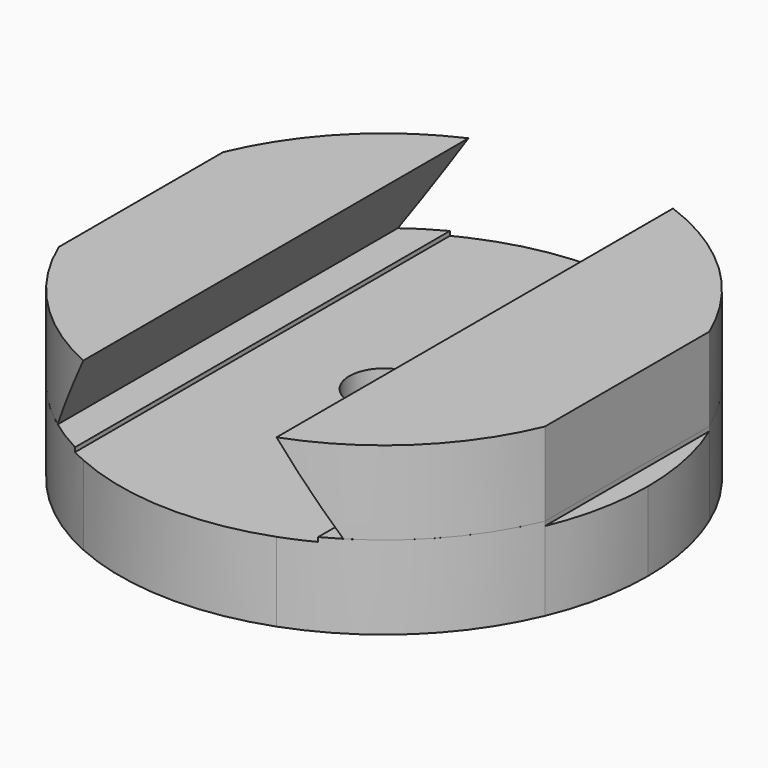
from build123d import *

# Parameters (mm, degrees)
F0_W          = 98.044
F0_H          = 98.044
F1_DEPTH      = 15.24
F3_D          = 12.7
F2_W          = 4.572
F2_H          = 98.044
F2_W_2        = 44.45
F4_DEPTH      = 0.7874
F6_DEPTH      = 50.8
F6_DEPTH_BACK = 50.8
F8_DEPTH      = 30.481
F10_DEPTH     = 30.481
F12_DEPTH     = 30.481


with BuildPart() as f1:
    # F0 (on Top) → F1 (new body)
    with BuildSketch(Plane.XY):
        Rectangle(F0_W, F0_H)
    extrude(amount=F1_DEPTH)

    # F3 (through all)
    with Locations(Plane.XY.offset(15.24)):
        with Locations((0, 0)):
            Hole(F3_D / 2)

    # F2 (on face) → F4 (cut)
    with BuildSketch(Plane.XY.offset(15.24)):
        with Locations((-46.736, 0)):
            Rectangle(F2_W, F2_H)
        with Locations((46.736, 0)):
            Rectangle(F2_W, F2_H)
        Rectangle(F2_W_2, F2_H)
    extrude(amount=-F4_DEPTH, mode=Mode.SUBTRACT)


with BuildPart() as f6:
    # F5 (on Front) → F6 (new body, two sides)
    with BuildSketch(Plane.XZ) as f6_sk:
        Polygon((-19.776182, 30.48), (-44.45, 30.48), (-44.45, 15.24), (-28.575, 15.24), align=None)
    extrude(amount=F6_DEPTH)
    extrude(f6_sk.sketch, amount=-F6_DEPTH_BACK)


with BuildPart() as f6b:
    # F5 (on Front) → F6, piece 2 (new body, two sides)
    with BuildSketch(Plane.XZ) as f6_2_sk:
        Polygon((25.4, 15.24), (44.45, 15.24), (44.45, 30.48), (16.601182, 30.48), align=None)
    extrude(amount=F6_DEPTH)
    extrude(f6_2_sk.sketch, amount=-F6_DEPTH_BACK)


with BuildPart() as f8_tool:
    # F7 (on face) → F8 (new body, through all)
    with BuildSketch(Plane.XY.offset(30.48)):
        with BuildLine():
            ThreePointArc((-44.45, 18.794284), (-34.501582, 33.744162), (-19.776182, 44.021929))
            Line((-19.776182, 44.021929), (-19.776182, 50.8))
            Line((-19.776182, 50.8), (-44.45, 50.8))
            Line((-44.45, 50.8), (-44.45, 18.794284))
        make_face()
        with BuildLine():
            Line((-19.776182, -50.8), (-19.776182, -44.021929))
            ThreePointArc((-19.776182, -44.021929), (-34.501582, -33.744162), (-44.45, -18.794284))
            Line((-44.45, -18.794284), (-44.45, -50.8))
            Line((-44.45, -50.8), (-19.776182, -50.8))
        make_face()
    extrude(amount=-F8_DEPTH)


with BuildPart() as f1_1:
    add(f1.part)

    # F8: cut by f8_tool
    add(f8_tool.part, mode=Mode.SUBTRACT)


with BuildPart() as f6_1:
    add(f6.part)

    # F8: cut by f8_tool
    add(f8_tool.part, mode=Mode.SUBTRACT)


with BuildPart() as f10_tool:
    # F9 (on face) → F10 (new body, through all)
    with BuildSketch(Plane.XY.offset(30.48)):
        with BuildLine():
            ThreePointArc((16.601182, 45.31477), (33.281312, 34.948274), (44.45, 18.794284))
            Line((44.45, 18.794284), (44.45, 50.8))
            Line((44.45, 50.8), (16.601182, 50.8))
            Line((16.601182, 50.8), (16.601182, 45.31477))
        make_face()
        with BuildLine():
            Line((44.45, -50.8), (44.45, -18.794284))
            ThreePointArc((44.45, -18.794284), (33.281312, -34.948274), (16.601182, -45.31477))
            Line((16.601182, -45.31477), (16.601182, -50.8))
            Line((16.601182, -50.8), (44.45, -50.8))
        make_face()
    extrude(amount=-F10_DEPTH)


with BuildPart() as f1_2:
    add(f1_1.part)

    # F10: cut by f10_tool
    add(f10_tool.part, mode=Mode.SUBTRACT)

    # F11 (on face) → F12 (cut, through all)
    with BuildSketch(Plane(origin=(0, 0, 0), x_dir=(1, 0, 0), z_dir=(0, 0, -1))):
        with BuildLine():
            ThreePointArc((-19.776182, 44.021929), (-1.714064, 48.229551), (16.601182, 45.31477))
            Line((16.601182, 45.31477), (16.601182, 49.022))
            Line((16.601182, 49.022), (-19.776182, 49.022))
            Line((-19.776182, 49.022), (-19.776182, 44.021929))
        make_face()
        with BuildLine():
            ThreePointArc((-44.45, -18.794284), (-48.26, 0), (-44.45, 18.794284))
            Line((-44.45, 18.794284), (-44.45, 49.022))
            Line((-44.45, 49.022), (-49.022, 49.022))
            Line((-49.022, 49.022), (-49.022, -49.022))
            Line((-49.022, -49.022), (-44.45, -49.022))
            Line((-44.45, -49.022), (-44.45, -18.794284))
        make_face()
        with BuildLine():
            Line((16.601182, -49.022), (16.601182, -45.31477))
            ThreePointArc((16.601182, -45.31477), (-1.714064, -48.229551), (-19.776182, -44.021929))
            Line((-19.776182, -44.021929), (-19.776182, -49.022))
            Line((-19.776182, -49.022), (16.601182, -49.022))
        make_face()
        with BuildLine():
            ThreePointArc((44.45, 18.794284), (47.29791, 9.58829), (48.26, 0))
            ThreePointArc((48.26, 0), (47.29791, -9.58829), (44.45, -18.794284))
            Line((44.45, -18.794284), (44.45, -49.022))
            Line((44.45, -49.022), (49.022, -49.022))
            Line((49.022, -49.022), (49.022, 49.022))
            Line((49.022, 49.022), (44.45, 49.022))
            Line((44.45, 49.022), (44.45, 18.794284))
        make_face()
    extrude(amount=-F12_DEPTH, mode=Mode.SUBTRACT)


with BuildPart() as f6b_1:
    add(f6b.part)

    # F10: cut by f10_tool
    add(f10_tool.part, mode=Mode.SUBTRACT)


solid = Compound([f6_1.part, f1_2.part, f6b_1.part])
